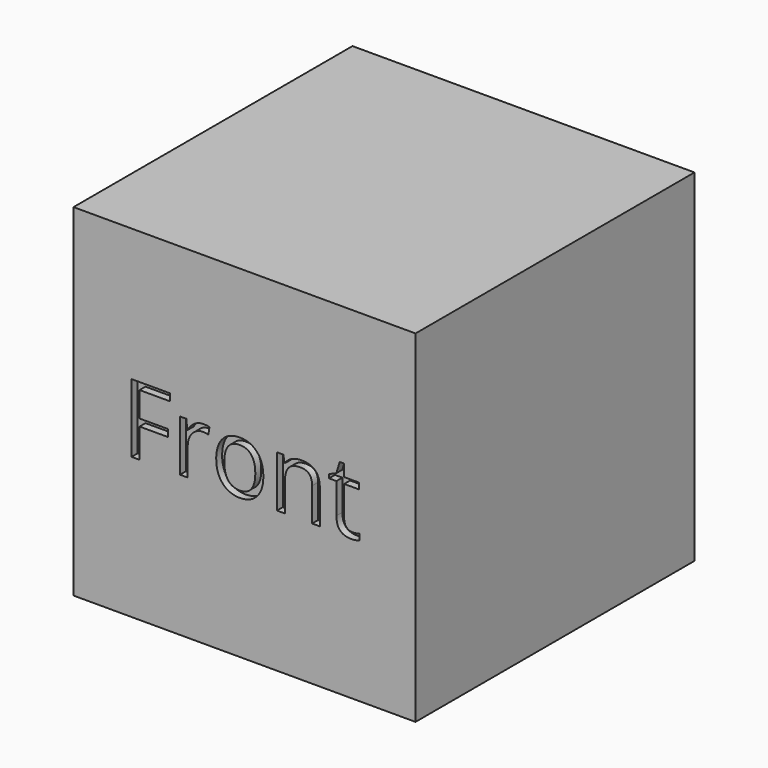
from build123d import *

# Parameters (mm, degrees)
F0_W         = 23.4188
F0_H         = 23.4188
F1_DEPTH     = 23.876
F2_TEXT_SIZE = 6.566071857
F3_DEPTH     = 0.508


# Not quite as in the source:
# - Text() gives the source's letters only with a copy of the font that has no kerning and outlines rounded to 1/6400 em; it was checked with that copy


with BuildPart() as f1:
    # F0 (on Front) → F1 (new body)
    with BuildSketch(Plane.XZ):
        Rectangle(F0_W, F0_H)
    extrude(amount=F1_DEPTH)

    # F2 (on face) → F3 (cut)
    with BuildSketch(Plane.XZ.offset(23.876)):
        with Locations((-8.3776194974, -2.0532531562)):
            Text('Front', F2_TEXT_SIZE, font='Open Sans', text_align=(TextAlign.LEFT, TextAlign.BOTTOM))
    extrude(amount=-F3_DEPTH, mode=Mode.SUBTRACT)


solid = f1.part
